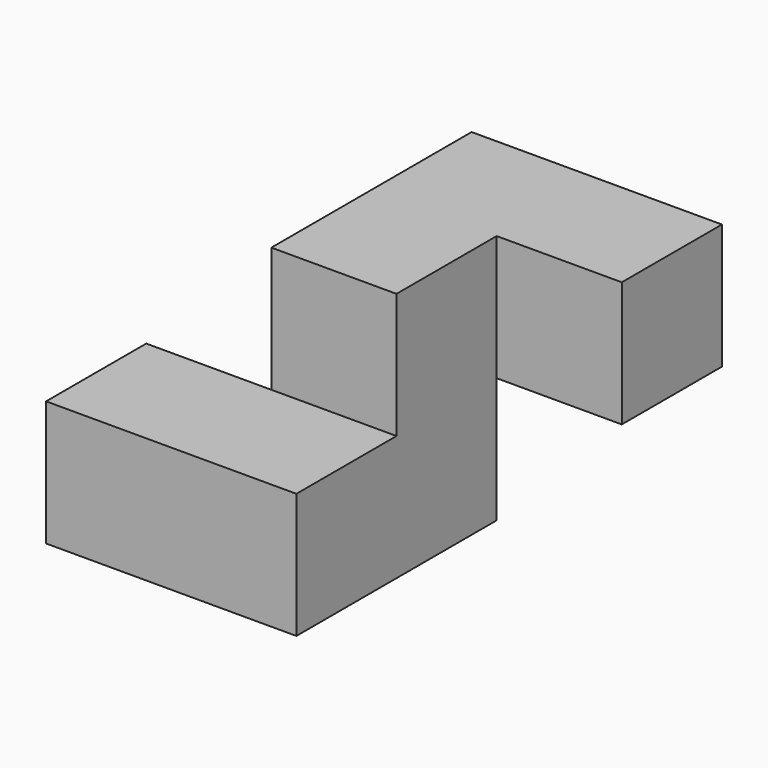
from build123d import *

# Parameters (mm, degrees)
F1_W      = 152.4
F1_H      = 76.2
F2_DEPTH  = 38.1
F3_W      = 76.2
F3_H      = 76.2
F4_DEPTH  = 76.2
F5_W      = 76.2
F5_H      = 76.2
F6_DEPTH  = 76.2
F7_W      = 76.2
F7_H      = 76.2
F8_DEPTH  = 76.2
F9_W      = 76.2
F9_H      = 76.2
F10_DEPTH = 76.2


# Not quite as in the source:
# - a variable given as a bare number and used for a length is read in inches; the dataset says mm whatever the document's units were


with BuildPart() as f2:
    # F1 (on Front) → F2 (new body, symmetric)
    with BuildSketch(Plane.XZ):
        Rectangle(F1_W, F1_H)
    extrude(amount=F2_DEPTH, both=True)

    # F3 (on face) → F4 (join)
    with BuildSketch(Plane(origin=(0, 38.1, 0), x_dir=(-1, 0, 0), z_dir=(0, 1, 0))):
        with Locations((-38.1, 0)):
            Rectangle(F3_W, F3_H)
    extrude(amount=F4_DEPTH)

    # F5 (on face) → F6 (join)
    with BuildSketch(Plane.XY.offset(38.1)):
        with Locations((38.1, 76.2)):
            Rectangle(F5_W, F5_H)
    extrude(amount=F6_DEPTH)

    # F7 (on face) → F8 (join)
    with BuildSketch(Plane(origin=(0, 114.3, 0), x_dir=(-1, 0, 0), z_dir=(0, 1, 0))):
        with Locations((-38.1, 76.2)):
            Rectangle(F7_W, F7_H)
    extrude(amount=F8_DEPTH)

    # F9 (on face) → F10 (join)
    with BuildSketch(Plane.YZ.offset(76.2)):
        with Locations((152.4, 76.2)):
            Rectangle(F9_W, F9_H)
    extrude(amount=F10_DEPTH)


solid = f2.part
